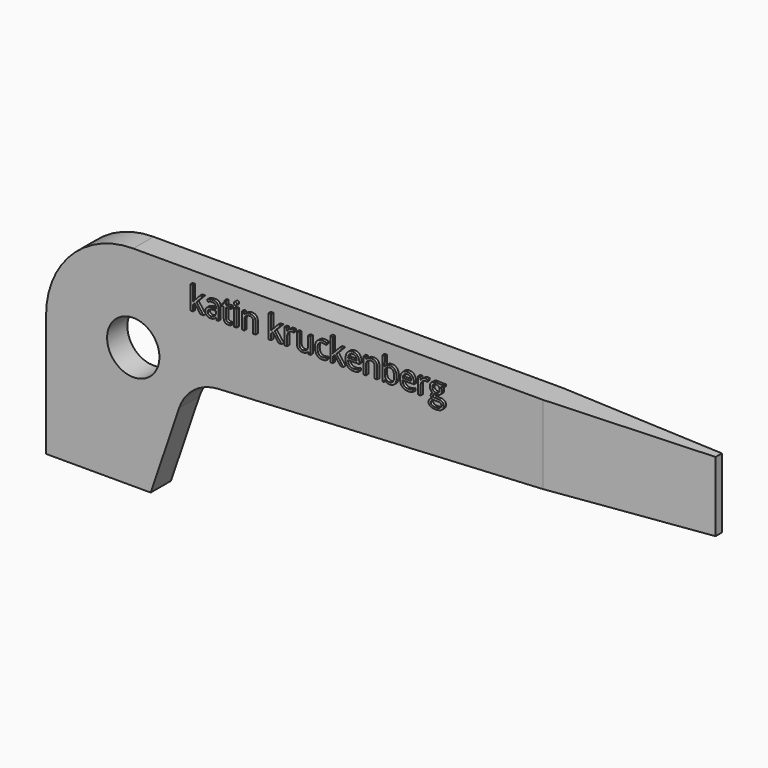
from build123d import *

# Parameters (mm, degrees)
F1_DEPTH     = 2.3090909091
F2_R         = 2.38125
F3_DEPTH     = 2.3100909091
F5_DEPTH     = 25.4
F6_TEXT_SIZE = 2.7802307159
F7_DEPTH     = 0.254


# Not quite as in the source:
# - Text() gives the source's letters only with a copy of the font that has no kerning and outlines rounded to 1/6400 em; it was checked with that copy


with BuildPart() as f1:
    # F0 (on Front) → F1 (new body)
    with BuildSketch(Plane.XZ):
        with BuildLine():
            Line((60.325, 19.05), (7.9375, 19.05))
            ThreePointArc((7.9375, 19.05), (2.3248399243, 16.7251600757), (0, 11.1125))
            Line((0, 11.1125), (0, 0))
            Line((0, 0), (9.525, 0))
            Line((9.525, 0), (12.1173647876, 7.6271664624))
            ThreePointArc((12.1173647876, 7.6271664624), (13.4786145605, 9.5135918491), (15.6631963617, 10.3130942181))
            Line((15.6631963617, 10.3130942181), (60.325, 12.7))
            Line((60.325, 12.7), (60.325, 19.05))
        make_face()
    extrude(amount=F1_DEPTH)

    # F2 (on face) → F3 (cut, through all)
    with BuildSketch(Plane.XZ.offset(2.3090909091)):
        with Locations((7.9375, 11.1125)):
            Circle(F2_R)
    extrude(amount=-F3_DEPTH, mode=Mode.SUBTRACT)

    # F4 (on face) → F5 (cut)
    with BuildSketch(Plane.XY.offset(19.05)):
        Polygon((60.325, 0), (45.24375, 0), (60.325, -0.79375), align=None)
        Polygon((60.325, -2.3090909091), (60.325, -1.5153409091), (45.24375, -2.3090909091), align=None)
    extrude(amount=-F5_DEPTH, mode=Mode.SUBTRACT)

    # F6 (on face) → F7 (join)
    with BuildSketch(Plane.XZ.offset(2.3090909091)):
        with Locations((13.1081482396, 15.9359946847)):
            Text('katin kruckenberg', F6_TEXT_SIZE, font='Open Sans', text_align=(TextAlign.LEFT, TextAlign.BOTTOM))
    extrude(amount=F7_DEPTH)


solid = f1.part
